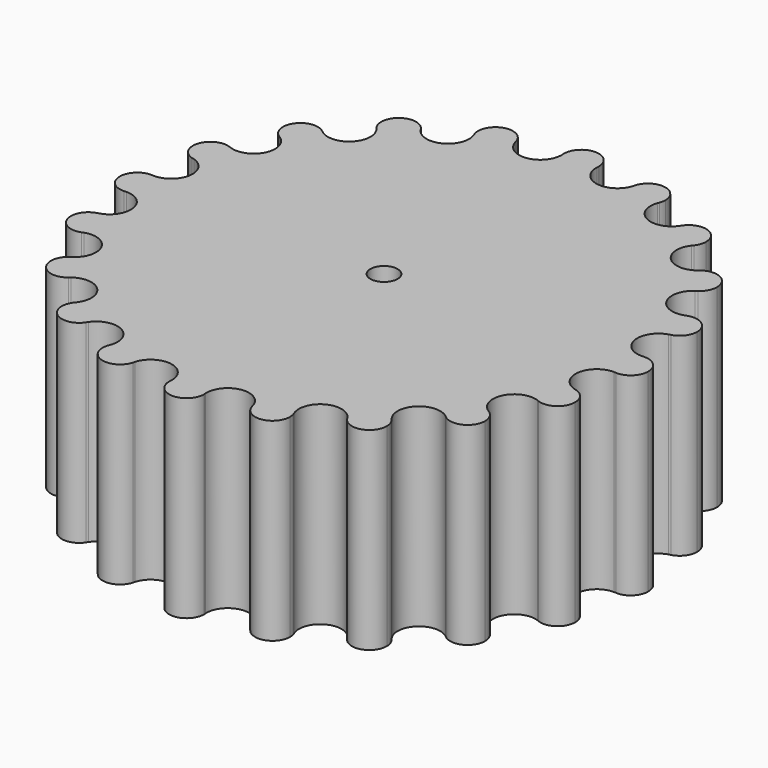
from build123d import *

# Parameters (mm, degrees)
F1_DEPTH = 25
F2_D     = 3.5


# Not quite as in the source:
# - ends of sketch curves that miss each other by under 0.0002 mm in the source are joined


with BuildPart() as f1:
    # F0 (on Top) → F1 (new body)
    with BuildSketch(Plane.XY):
        with BuildLine():
            ThreePointArc((2.2296111501, 31.5287732655), (2.2355164002, 31.6403797371), (2.245951629, 31.751654094))
            ThreePointArc((2.245951629, 31.751654094), (-0.0013246403, 31.8309885908), (-2.2485942989, 31.7514670543))
            ThreePointArc((-2.2485942989, 31.7514670543), (-2.239253826, 31.6547086385), (-2.2333389133, 31.5576805536))
            ThreePointArc((-2.2333389133, 31.5576805536), (-0.0145733277, 29.5810358148), (2.2296111501, 31.5287732655))
        make_face()
        with BuildLine():
            ThreePointArc((-2.2485942989, 31.7514670543), (-0.0013246403, 31.8309885908), (2.245951629, 31.751654094))
            ThreePointArc((2.245951629, 31.751654094), (2.2472729659, 31.7515606016), (2.2485942989, 31.7514670543))
            ThreePointArc((2.2485942989, 31.7514670543), (2.2496485473, 31.7912216247), (2.25, 31.8309886184))
            ThreePointArc((2.25, 31.8309886184), (-0.0397669937, 34.0806371656), (-2.2485942989, 31.7514670543))
        make_face()
        with BuildLine():
            ThreePointArc((7.6388793133, 30.7442870179), (4.5834620848, 28.7177750463), (2.2296111501, 31.5287732655))
            ThreePointArc((2.2296111501, 31.5287732655), (-0.0145733277, 29.5810358148), (-2.2333389133, 31.5576805536))
            ThreePointArc((-2.2333389133, 31.5576805536), (-4.5505150488, 28.7227559932), (-7.6304110311, 30.702741661))
            ThreePointArc((-7.6304110311, 30.702741661), (-7.5992731862, 30.4885414472), (-7.5888617869, 30.272340384))
            ThreePointArc((-7.5888617869, 30.272340384), (-9.3380350766, 28.0787878758), (-11.8659041036, 29.2958162182))
            ThreePointArc((-11.8659041036, 29.2958162182), (-13.2351692804, 25.8949542762), (-16.7673551666, 26.87699905))
            ThreePointArc((-16.7673551666, 26.87699905), (-16.5415521796, 26.3332821419), (-16.4645266095, 25.7496023266))
            ThreePointArc((-16.4645266095, 25.7496023266), (-17.8664108747, 23.6655678498), (-20.3251485654, 24.178489054))
            ThreePointArc((-20.3251485654, 24.178489054), (-20.6525550241, 20.478008628), (-24.3674905167, 20.4801670487))
            ThreePointArc((-24.3674905167, 20.4801670487), (-24.3689908678, 20.4783817844), (-24.3704910882, 20.4765964102))
            ThreePointArc((-24.3704910882, 20.4765964102), (-23.7352137216, 19.6904266331), (-23.5081825547, 18.705491559))
            ThreePointArc((-23.5081825547, 18.705491559), (-24.5875207675, 16.7840205132), (-26.7900056481, 16.7060313559))
            ThreePointArc((-26.7900056481, 16.7060313559), (-25.9733845183, 13.0874478649), (-29.5035803073, 11.9478276466))
            ThreePointArc((-29.5035803073, 11.9478276466), (-29.5047483027, 11.9449430312), (-29.505916016, 11.9420583017))
            ThreePointArc((-29.505916016, 11.9420583017), (-28.4357647794, 11.1179502524), (-28.0303475025, 9.8295347225))
            ThreePointArc((-28.0303475025, 9.8295347225), (-28.8194745011, 8.1182924621), (-30.6333253458, 7.6073946184))
            ThreePointArc((-30.6333253458, 7.6073946184), (-28.7472439398, 4.4166259857), (-31.751654094, 2.245951629))
            ThreePointArc((-31.751654094, 2.245951629), (-31.7519025839, 2.2424358908), (-31.7521506846, 2.2389201252))
            ThreePointArc((-31.7521506846, 2.2389201252), (-30.2171769295, 1.5507851285), (-29.58836044, -0.0094276855))
            ThreePointArc((-29.58836044, -0.0094276855), (-30.1261933213, -1.4692166284), (-31.4825682246, -2.2311189106))
            ThreePointArc((-31.4825682246, -2.2311189106), (-28.7049434665, -4.6840543352), (-30.8916547511, -7.6757737825))
            ThreePointArc((-30.8916547511, -7.6757737825), (-30.8908035046, -7.6791988688), (-30.8899518782, -7.6826238607))
            ThreePointArc((-30.8899518782, -7.6826238607), (-28.9215036913, -8.0544752034), (-28.0297122057, -9.8482894724))
            ThreePointArc((-28.0297122057, -9.8482894724), (-28.36051631, -11.0226774466), (-29.2556563069, -11.8517388769))
            ThreePointArc((-29.2556563069, -11.8517388769), (-25.8533101031, -13.3234724767), (-27.0077650064, -16.8461409759))
            ThreePointArc((-27.0077650064, -16.8461409759), (-27.0061104746, -16.8487932345), (-27.0044556823, -16.8514453305))
            ThreePointArc((-27.0044556823, -16.8514453305), (-24.6949791981, -16.7403548583), (-23.5069741483, -18.7239542951))
            ThreePointArc((-23.5069741483, -18.7239542951), (-23.6790191272, -19.5868580732), (-24.1688434197, -20.3177989515))
            ThreePointArc((-24.1688434197, -20.3177989515), (-20.473920736, -20.6570330767), (-20.4801670487, -24.3674905167))
            ThreePointArc((-20.4801670487, -24.3674905167), (-20.4783650945, -24.3690048931), (-20.4765630283, -24.3705191362))
            ThreePointArc((-20.4765630283, -24.3705191362), (-17.9732094776, -23.6426603342), (-16.4628633807, -25.7676102403))
            ThreePointArc((-16.4628633807, -25.7676102403), (-16.5270410789, -26.3011651716), (-16.7159130383, -26.8042824787))
            ThreePointArc((-16.7159130383, -26.8042824787), (-13.1504393756, -25.9385454074), (-11.8979495568, -29.3872223087))
            ThreePointArc((-11.8979495568, -29.3872223087), (-9.3758462327, -28.0875210272), (-7.5869065441, -30.2897751881))
            ThreePointArc((-7.5869065441, -30.2897751881), (-7.5953497313, -30.484513615), (-7.6206159263, -30.6777905193))
            ThreePointArc((-7.6206159263, -30.6777905193), (-4.5254450945, -28.7268224726), (-2.2316153244, -31.5772090749))
            ThreePointArc((-2.2316153244, -31.5772090749), (-0.0074108445, -29.5978080409), (2.2333711069, -31.5584228089))
            ThreePointArc((2.2333711069, -31.5584228089), (4.5439992997, -28.7237961539), (7.6270501821, -30.6907501888))
            ThreePointArc((7.6270501821, -30.6907501888), (9.1696510411, -28.1416061572), (11.8894052748, -29.3584420593))
            ThreePointArc((11.8894052748, -29.3584420593), (13.1703633173, -25.9280084163), (16.7239937694, -26.8114330567))
            ThreePointArc((16.7239937694, -26.8114330567), (17.4895545067, -23.8804266566), (20.4793701707, -24.3681602473))
            ThreePointArc((20.4793701707, -24.3681602473), (20.480782657, -24.3669731026), (20.4821950744, -24.365785876))
            ThreePointArc((20.4821950744, -24.365785876), (20.4778391425, -20.6529170029), (24.1757312537, -20.3197381058))
            ThreePointArc((24.1757312537, -20.3197381058), (24.0164987851, -17.3003655793), (27.0061468011, -16.8487350083))
            ThreePointArc((27.0061468011, -16.8487350083), (27.0076570143, -16.8463141078), (27.0091670106, -16.843893072))
            ThreePointArc((27.0091670106, -16.843893072), (25.8549292547, -13.320187234), (29.2589931432, -11.8501135376))
            ThreePointArc((29.2589931432, -11.8501135376), (28.1870798883, -9.0265052707), (30.8905822169, -7.6800889791))
            ThreePointArc((30.8905822169, -7.6800889791), (30.8914380482, -7.6766458651), (30.8922934958, -7.6732026557))
            ThreePointArc((30.8922934958, -7.6732026557), (28.70523581, -4.682564819), (31.4809443082, -2.2284706228))
            ThreePointArc((31.4809443082, -2.2284706228), (29.5945431655, 0.1288406823), (31.7520116692, 2.2408907565))
            ThreePointArc((31.7520116692, 2.2408907565), (31.7517395954, 2.2447425442), (31.7514670543, 2.2485942989))
            ThreePointArc((31.7514670543, 2.2485942989), (28.7475271566, 4.4159083123), (30.6266181526, 7.6080740302))
            ThreePointArc((30.6266181526, 7.6080740302), (28.1034407528, 9.2681161095), (29.5054107708, 11.9433065635))
            ThreePointArc((29.5054107708, 11.9433065635), (29.5039984877, 11.9467949535), (29.5025857922, 11.9502831766))
            ThreePointArc((29.5025857922, 11.9502831766), (25.9750631091, 13.0847683856), (26.7794779087, 16.70186526))
            ThreePointArc((26.7794779087, 16.70186526), (23.8623879535, 17.4966801283), (24.3699852255, 20.4771984542))
            ThreePointArc((24.3699852255, 20.4771984542), (24.3678856788, 20.4796968719), (24.365785876, 20.4821950744))
            ThreePointArc((24.365785876, 20.4821950744), (20.6568603558, 20.4742463598), (20.3132875285, 24.1672328761))
            ThreePointArc((20.3132875285, 24.1672328761), (17.2888909502, 24.0104247691), (16.8479825647, 27.0066162249))
            ThreePointArc((16.8479825647, 27.0066162249), (16.8459378666, 27.0078916952), (16.843893072, 27.0091670106))
            ThreePointArc((16.843893072, 27.0091670106), (13.3119213441, 25.858669666), (11.8560873562, 29.2761271751))
            ThreePointArc((11.8560873562, 29.2761271751), (9.0992045072, 28.1480619772), (7.6388793133, 30.7442870179))
        make_face()
        with BuildLine():
            ThreePointArc((-7.6304110311, 30.702741661), (-7.6547612288, 30.7967974802), (-7.6757737825, 30.8916547511))
            ThreePointArc((-7.6757737825, 30.8916547511), (-9.8375762301, 30.272659783), (-11.9502831766, 29.5025857922))
            ThreePointArc((-11.9502831766, 29.5025857922), (-11.9059938401, 29.4000578971), (-11.8659041036, 29.2958162182))
            ThreePointArc((-11.8659041036, 29.2958162182), (-9.3380350766, 28.0787878758), (-7.5888617869, 30.272340384))
            ThreePointArc((-7.5888617869, 30.272340384), (-7.5992731862, 30.4885414472), (-7.6304110311, 30.702741661))
        make_face()
        with BuildLine():
            ThreePointArc((-11.9502831766, 29.5025857922), (-9.8375762301, 30.272659783), (-7.6757737825, 30.8916547511))
            ThreePointArc((-7.6757737825, 30.8916547511), (-10.5343279004, 32.412159742), (-11.9527324859, 29.5015935594))
            ThreePointArc((-11.9527324859, 29.5015935594), (-11.9515078415, 29.5020897012), (-11.9502831766, 29.5025857922))
        make_face()
        with BuildLine():
            ThreePointArc((7.6645571269, 30.8513022958), (7.652253607, 30.7976661933), (7.6388793133, 30.7442870179))
            ThreePointArc((7.6388793133, 30.7442870179), (9.0992045072, 28.1480619772), (11.8560873562, 29.2761271751))
            ThreePointArc((11.8560873562, 29.2761271751), (11.8994205773, 29.3908769768), (11.9478276466, 29.5035803073))
            ThreePointArc((11.9478276466, 29.5035803073), (9.8362792973, 30.273081211), (7.675697998, 30.8916735815))
            ThreePointArc((7.675697998, 30.8916735815), (7.6700336292, 30.8715138605), (7.6645571269, 30.8513022958))
        make_face()
        with BuildLine():
            ThreePointArc((12.088962408, 30.2729756809), (10.1513364446, 32.5011862771), (7.675697998, 30.8916735815))
            ThreePointArc((7.675697998, 30.8916735815), (9.8362792973, 30.273081211), (11.9478276466, 29.5035803073))
            ThreePointArc((11.9478276466, 29.5035803073), (11.9502229883, 29.5026101719), (11.9526182512, 29.5016398419))
            ThreePointArc((11.9526182512, 29.5016398419), (12.054614191, 29.8813289314), (12.088962408, 30.2729756809))
        make_face()
        with BuildLine():
            ThreePointArc((-16.4645266095, 25.7496023266), (-16.5415521796, 26.3332821419), (-16.7673551666, 26.87699905))
            ThreePointArc((-16.7673551666, 26.87699905), (-16.7970480412, 26.9243760458), (-16.8257715617, 26.9723469318))
            ThreePointArc((-16.8257715617, 26.9723469318), (-16.8369478592, 26.9894402339), (-16.8482788472, 27.0064313879))
            ThreePointArc((-16.8482788472, 27.0064313879), (-18.7118765222, 25.7502915215), (-20.4821950744, 24.365785876))
            ThreePointArc((-20.4821950744, 24.365785876), (-20.401589879, 24.2738831516), (-20.3251485654, 24.178489054))
            ThreePointArc((-20.3251485654, 24.178489054), (-17.8664108747, 23.6655678498), (-16.4645266095, 25.7496023266))
        make_face()
        with BuildLine():
            ThreePointArc((-20.4821950744, 24.365785876), (-18.7118765222, 25.7502915215), (-16.8482788472, 27.0064313879))
            ThreePointArc((-16.8482788472, 27.0064313879), (-20.0373369692, 27.569677257), (-20.4860970483, 24.362505293))
            ThreePointArc((-20.4860970483, 24.362505293), (-20.484146127, 24.3641456626), (-20.4821950744, 24.365785876))
        make_face()
        with BuildLine():
            ThreePointArc((20.9649192446, 25.7508107331), (19.3713841981, 27.9029152298), (16.8479825647, 27.0066162249))
            ThreePointArc((16.8479825647, 27.0066162249), (18.7106636579, 25.7511728258), (20.4801670487, 24.3674905167))
            ThreePointArc((20.4801670487, 24.3674905167), (20.4829651807, 24.365138494), (20.4857630425, 24.36278615))
            ThreePointArc((20.4857630425, 24.36278615), (20.8417594531, 25.0166099926), (20.9649192446, 25.7508107331))
        make_face()
        with BuildLine():
            ThreePointArc((20.4801670487, 24.3674905167), (18.7106636579, 25.7511728258), (16.8479825647, 27.0066162249))
            ThreePointArc((16.8479825647, 27.0066162249), (17.2888909502, 24.0104247691), (20.3132875285, 24.1672328761))
            ThreePointArc((20.3132875285, 24.1672328761), (20.3943531214, 24.2693401472), (20.4801670487, 24.3674905167))
        make_face()
        with BuildLine():
            ThreePointArc((-23.5081825547, 18.705491559), (-23.7352137216, 19.6904266331), (-24.3704910882, 20.4765964102))
            ThreePointArc((-24.3704910882, 20.4765964102), (-25.7539598891, 18.7068272685), (-27.0091670106, 16.843893072))
            ThreePointArc((-27.0091670106, 16.843893072), (-26.8979629467, 16.7775429358), (-26.7900056481, 16.7060313559))
            ThreePointArc((-26.7900056481, 16.7060313559), (-24.5875207675, 16.7840205132), (-23.5081825547, 18.705491559))
        make_face()
        with BuildLine():
            ThreePointArc((-27.0091670106, 16.843893072), (-25.7539598891, 18.7068272685), (-24.3704910882, 20.4765964102))
            ThreePointArc((-24.3704910882, 20.4765964102), (-27.5787706675, 20.0275955352), (-27.0129361537, 16.8378477478))
            ThreePointArc((-27.0129361537, 16.8378477478), (-27.0110517513, 16.8408705153), (-27.0091670106, 16.843893072))
        make_face()
        with BuildLine():
            ThreePointArc((28.0090300121, 18.7071547879), (26.7431918967, 20.7304998857), (24.3699852255, 20.4771984542))
            ThreePointArc((24.3699852255, 20.4771984542), (25.7529503033, 18.708217101), (27.0077650064, 16.8461409759))
            ThreePointArc((27.0077650064, 16.8461409759), (27.0101103939, 16.8423802632), (27.0124552578, 16.838619224))
            ThreePointArc((27.0124552578, 16.838619224), (27.7443142239, 17.6483126851), (28.0090300121, 18.7071547879))
        make_face()
        with BuildLine():
            ThreePointArc((27.0077650064, 16.8461409759), (25.7529503033, 18.708217101), (24.3699852255, 20.4771984542))
            ThreePointArc((24.3699852255, 20.4771984542), (23.8623879535, 17.4966801283), (26.7794779087, 16.70186526))
            ThreePointArc((26.7794779087, 16.70186526), (26.8918493622, 16.7768071), (27.0077650064, 16.8461409759))
        make_face()
        with BuildLine():
            ThreePointArc((-28.0303475025, 9.8295347225), (-28.4357647794, 11.1179502524), (-29.505916016, 11.9420583017))
            ThreePointArc((-29.505916016, 11.9420583017), (-30.2744398823, 9.8320967365), (-30.8922934958, 7.6732026557))
            ThreePointArc((-30.8922934958, 7.6732026557), (-30.7620096837, 7.6434457669), (-30.6333253458, 7.6073946184))
            ThreePointArc((-30.6333253458, 7.6073946184), (-28.8194745011, 8.1182924621), (-28.0303475025, 9.8295347225))
        make_face()
        with BuildLine():
            ThreePointArc((-30.8922934958, 7.6732026557), (-30.2744398823, 9.8320967365), (-29.505916016, 11.9420583017))
            ThreePointArc((-29.505916016, 11.9420583017), (-32.4204145672, 10.5242382267), (-30.8943466392, 7.6649319737))
            ThreePointArc((-30.8943466392, 7.6649319737), (-30.8933203443, 7.6690673834), (-30.8922934958, 7.6732026557))
        make_face()
        with BuildLine():
            ThreePointArc((32.5317680695, 9.8314899652), (31.5693425485, 11.6766598655), (29.5054107708, 11.9433065635))
            ThreePointArc((29.5054107708, 11.9433065635), (30.2738226844, 9.8339969747), (30.8916547511, 7.6757737825))
            ThreePointArc((30.8916547511, 7.6757737825), (30.892821041, 7.6710784476), (30.8939866173, 7.6663829356))
            ThreePointArc((30.8939866173, 7.6663829356), (32.0762027622, 8.4741012465), (32.5317680695, 9.8314899652))
        make_face()
        with BuildLine():
            ThreePointArc((30.8916547511, 7.6757737825), (30.2738226844, 9.8339969747), (29.5054107708, 11.9433065635))
            ThreePointArc((29.5054107708, 11.9433065635), (28.1034407528, 9.2681161095), (30.6266181526, 7.6080740302))
            ThreePointArc((30.6266181526, 7.6080740302), (30.7582941568, 7.6452213931), (30.8916547511, 7.6757737825))
        make_face()
        with BuildLine():
            ThreePointArc((-29.58836044, -0.0094276855), (-30.2171769295, 1.5507851285), (-31.7521506846, 2.2389201252))
            ThreePointArc((-31.7521506846, 2.2389201252), (-31.830988249, -0.0048491491), (-31.7514670543, -2.2485942989))
            ThreePointArc((-31.7514670543, -2.2485942989), (-31.6172318146, -2.2365610298), (-31.4825682246, -2.2311189106))
            ThreePointArc((-31.4825682246, -2.2311189106), (-30.1261933213, -1.4692166284), (-29.58836044, -0.0094276855))
        make_face()
        with BuildLine():
            ThreePointArc((-31.7514670543, -2.2485942989), (-31.830988249, -0.0048491491), (-31.7521506846, 2.2389201252))
            ThreePointArc((-31.7521506846, 2.2389201252), (-34.0883603414, -0.010093935), (-31.7508191792, -2.2577240467))
            ThreePointArc((-31.7508191792, -2.2577240467), (-31.7511434449, -2.2531591961), (-31.7514670543, -2.2485942989))
        make_face()
        with BuildLine():
            ThreePointArc((34.0904163039, -0.0073718217), (33.3998376023, 1.6145730646), (31.7520116692, 2.2408907565))
            ThreePointArc((31.7520116692, 2.2408907565), (31.8112382538, 1.1211410194), (31.8309886184, 0))
            ThreePointArc((31.8309886184, 0), (31.8111488043, -1.1236761863), (31.751654094, -2.245951629))
            ThreePointArc((31.751654094, -2.245951629), (31.7513127255, -2.2507724521), (31.7509706251, -2.2555932233))
            ThreePointArc((31.7509706251, -2.2555932233), (33.3994620413, -1.629677708), (34.0904163039, -0.0073718217))
        make_face()
        with BuildLine():
            ThreePointArc((31.8309886184, 0), (31.8112382538, 1.1211410194), (31.7520116692, 2.2408907565))
            ThreePointArc((31.7520116692, 2.2408907565), (29.5945431655, 0.1288406823), (31.4809443082, -2.2284706228))
            ThreePointArc((31.4809443082, -2.2284706228), (31.616514884, -2.2338710741), (31.751654094, -2.245951629))
            ThreePointArc((31.751654094, -2.245951629), (31.8111488043, -1.1236761863), (31.8309886184, 0))
        make_face()
        with BuildLine():
            ThreePointArc((-28.0297122057, -9.8482894724), (-28.9215036913, -8.0544752034), (-30.8899518782, -7.6826238607))
            ThreePointArc((-30.8899518782, -7.6826238607), (-30.2715688489, -9.8409326716), (-29.5025857922, -11.9502831766))
            ThreePointArc((-29.5025857922, -11.9502831766), (-29.3803126395, -11.8980251747), (-29.2556563069, -11.8517388769))
            ThreePointArc((-29.2556563069, -11.8517388769), (-28.36051631, -11.0226774466), (-28.0297122057, -9.8482894724))
        make_face()
        with BuildLine():
            ThreePointArc((-29.5025857922, -11.9502831766), (-30.2715688489, -9.8409326716), (-30.8899518782, -7.6826238607))
            ThreePointArc((-30.8899518782, -7.6826238607), (-32.419385451, -10.5442049869), (-29.4992227607, -11.9585823967))
            ThreePointArc((-29.4992227607, -11.9585823967), (-29.5009045683, -11.9544329049), (-29.5025857922, -11.9502831766))
        make_face()
        with BuildLine():
            ThreePointArc((32.5324033664, -9.8463342297), (32.0755712913, -8.487272497), (30.8905822169, -7.6800889791))
            ThreePointArc((30.8905822169, -7.6800889791), (30.2723820517, -9.8384308373), (29.5035803073, -11.9478276466))
            ThreePointArc((29.5035803073, -11.9478276466), (29.5019219736, -11.9519218658), (29.5002630717, -11.9560158548))
            ThreePointArc((29.5002630717, -11.9560158548), (31.5674489565, -11.6932662348), (32.5324033664, -9.8463342297))
        make_face()
        with BuildLine():
            ThreePointArc((29.5035803073, -11.9478276466), (30.2723820517, -9.8384308373), (30.8905822169, -7.6800889791))
            ThreePointArc((30.8905822169, -7.6800889791), (28.1870798883, -9.0265052707), (29.2589931432, -11.8501135376))
            ThreePointArc((29.2589931432, -11.8501135376), (29.3824572283, -11.8960407182), (29.5035803073, -11.9478276466))
        make_face()
        with BuildLine():
            ThreePointArc((-23.5069741483, -18.7239542951), (-24.6949791981, -16.7403548583), (-27.0044556823, -16.8514453305))
            ThreePointArc((-27.0044556823, -16.8514453305), (-25.7491944605, -18.7133861462), (-24.365785876, -20.4821950744))
            ThreePointArc((-24.365785876, -20.4821950744), (-24.2692326947, -20.3976992406), (-24.1688434197, -20.3177989515))
            ThreePointArc((-24.1688434197, -20.3177989515), (-23.6790191272, -19.5868580732), (-23.5069741483, -18.7239542951))
        make_face()
        with BuildLine():
            ThreePointArc((-24.365785876, -20.4821950744), (-25.7491944605, -18.7133861462), (-27.0044556823, -16.8514453305))
            ThreePointArc((-27.0044556823, -16.8514453305), (-27.5769123054, -20.0469528227), (-24.3606712048, -20.4882779871))
            ThreePointArc((-24.3606712048, -20.4882779871), (-24.3632287303, -20.4852366904), (-24.365785876, -20.4821950744))
        make_face()
        with BuildLine():
            ThreePointArc((28.0102384186, -18.7222910663), (27.7433916982, -17.6594632017), (27.0061468011, -16.8487350083))
            ThreePointArc((27.0061468011, -16.8487350083), (25.7509121679, -18.7110223917), (24.3674905167, -20.4801670487))
            ThreePointArc((24.3674905167, -20.4801670487), (24.365153247, -20.4829476315), (24.3628156601, -20.4857279474))
            ThreePointArc((24.3628156601, -20.4857279474), (26.7396001478, -20.747963943), (28.0102384186, -18.7222910663))
        make_face()
        with BuildLine():
            ThreePointArc((24.3674905167, -20.4801670487), (25.7509121679, -18.7110223917), (27.0061468011, -16.8487350083))
            ThreePointArc((27.0061468011, -16.8487350083), (24.0164987851, -17.3003655793), (24.1757312537, -20.3197381058))
            ThreePointArc((24.1757312537, -20.3197381058), (24.2734350163, -20.3977722098), (24.3674905167, -20.4801670487))
        make_face()
        with BuildLine():
            ThreePointArc((-16.4628633807, -25.7676102403), (-17.9732094776, -23.6426603342), (-20.4765630283, -24.3705191362))
            ThreePointArc((-20.4765630283, -24.3705191362), (-18.70680963, -25.7539727011), (-16.843893072, -27.0091670106))
            ThreePointArc((-16.843893072, -27.0091670106), (-16.782153876, -26.9053187813), (-16.7159130383, -26.8042824787))
            ThreePointArc((-16.7159130383, -26.8042824787), (-16.5270410789, -26.3011651716), (-16.4628633807, -25.7676102403))
        make_face()
        with BuildLine():
            ThreePointArc((-16.843893072, -27.0091670106), (-18.70680963, -25.7539727011), (-20.4765630283, -24.3705191362))
            ThreePointArc((-20.4765630283, -24.3705191362), (-20.0349916644, -27.5881807007), (-16.8386060698, -27.0124634576))
            ThreePointArc((-16.8386060698, -27.0124634576), (-16.8412496516, -27.0108153634), (-16.843893072, -27.0091670106))
        make_face()
        with BuildLine():
            ThreePointArc((20.9665824734, -25.7664018338), (20.8412909615, -25.0260547256), (20.4793701707, -24.3681602473))
            ThreePointArc((20.4793701707, -24.3681602473), (18.7093646047, -25.7521166608), (16.8461409759, -27.0077650064))
            ThreePointArc((16.8461409759, -27.0077650064), (16.8439724694, -27.0091174953), (16.8418038543, -27.01046981))
            ThreePointArc((16.8418038543, -27.01046981), (19.3662932194, -27.9205550193), (20.9665824734, -25.7664018338))
        make_face()
        with BuildLine():
            ThreePointArc((16.8461409759, -27.0077650064), (18.7093646047, -25.7521166608), (20.4793701707, -24.3681602473))
            ThreePointArc((20.4793701707, -24.3681602473), (17.4895545067, -23.8804266566), (16.7239937694, -26.8114330567))
            ThreePointArc((16.7239937694, -26.8114330567), (16.7871318014, -26.9083146548), (16.8461409759, -27.0077650064))
        make_face()
        with BuildLine():
            ThreePointArc((11.9421871063, -29.4846731889), (11.9150110155, -29.4218859344), (11.8894052748, -29.3584420593))
            ThreePointArc((11.8894052748, -29.3584420593), (9.1696510411, -28.1416061572), (7.6270501821, -30.6907501888))
            ThreePointArc((7.6270501821, -30.6907501888), (7.6533004986, -30.7907444649), (7.6757737825, -30.8916547511))
            ThreePointArc((7.6757737825, -30.8916547511), (9.8369854282, -30.272851767), (11.9491316249, -29.5030522122))
            ThreePointArc((11.9491316249, -29.5030522122), (11.9456794267, -29.4938551205), (11.9421871063, -29.4846731889))
        make_face()
        with BuildLine():
            ThreePointArc((-7.5869065441, -30.2897751881), (-9.3758462327, -28.0875210272), (-11.8979495568, -29.3872223087))
            ThreePointArc((-11.8979495568, -29.3872223087), (-11.9124043492, -29.422499831), (-11.9273468036, -29.457573577))
            ThreePointArc((-11.9273468036, -29.457573577), (-11.9365251305, -29.4810095904), (-11.9454407246, -29.5045468075))
            ThreePointArc((-11.9454407246, -29.5045468075), (-9.8338320221, -30.2738762663), (-7.6732026557, -30.8922934958))
            ThreePointArc((-7.6732026557, -30.8922934958), (-7.649063525, -30.7845138837), (-7.6206159263, -30.6777905193))
            ThreePointArc((-7.6206159263, -30.6777905193), (-7.5953497313, -30.484513615), (-7.5869065441, -30.2897751881))
        make_face()
        with BuildLine():
            ThreePointArc((-7.6732026557, -30.8922934958), (-9.8338320221, -30.2738762663), (-11.9454407246, -29.5045468075))
            ThreePointArc((-11.9454407246, -29.5045468075), (-10.5318856077, -32.4297527817), (-7.6693464279, -30.8932510719))
            ThreePointArc((-7.6693464279, -30.8932510719), (-7.6712745567, -30.892772344), (-7.6732026557, -30.8922934958))
        make_face()
        with BuildLine():
            ThreePointArc((12.0909176508, -30.2891398912), (12.0551874448, -29.8897537634), (11.9491316249, -29.5030522122))
            ThreePointArc((11.9491316249, -29.5030522122), (9.8369854282, -30.272851767), (7.6757737825, -30.8916547511))
            ThreePointArc((7.6757737825, -30.8916547511), (7.6745187077, -30.8919665775), (7.6732636203, -30.892278353))
            ThreePointArc((7.6732636203, -30.892278353), (10.1452845604, -32.5184583486), (12.0909176508, -30.2891398912))
        make_face()
        with BuildLine():
            ThreePointArc((2.2485942989, -31.7514670543), (2.2392830044, -31.6550789674), (2.2333711069, -31.5584228089))
            ThreePointArc((2.2333711069, -31.5584228089), (-0.0074108445, -29.5978080409), (-2.2316153244, -31.5772090749))
            ThreePointArc((-2.2316153244, -31.5772090749), (-2.2373952316, -31.6645456737), (-2.245951629, -31.751654094))
            ThreePointArc((-2.245951629, -31.751654094), (0.0013246403, -31.8309885908), (2.2485942989, -31.7514670543))
        make_face()
        with BuildLine():
            ThreePointArc((2.2485942989, -31.7514670543), (0.0013246403, -31.8309885908), (-2.245951629, -31.751654094))
            ThreePointArc((-2.245951629, -31.751654094), (-0.0460208017, -34.0972744301), (2.2520558639, -31.8477881256))
            ThreePointArc((2.2520558639, -31.8477881256), (2.2515390788, -31.7995671151), (2.2499889609, -31.7513682555))
            ThreePointArc((2.2499889609, -31.7513682555), (2.2492916304, -31.7514176626), (2.2485942989, -31.7514670543))
        make_face()
    extrude(amount=F1_DEPTH)

    # F2 (through all)
    with Locations(Plane(origin=(0, 0, 0), x_dir=(1, 0, 0), z_dir=(0, 0, -1))):
        with Locations((0.0010279319, 0.0083997536)):
            Hole(F2_D / 2)


solid = f1.part
